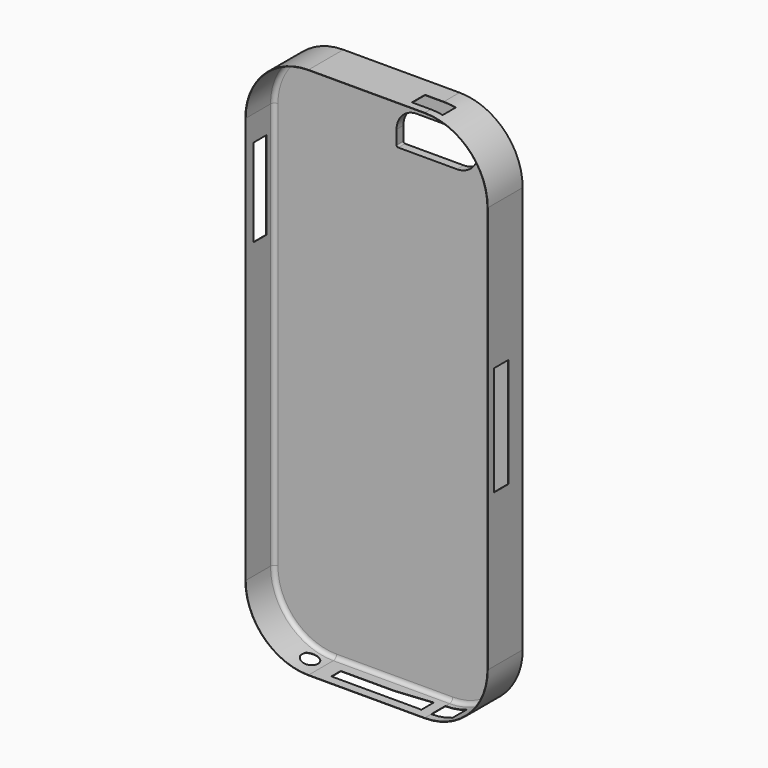
from build123d import *

# Parameters (mm, degrees)
F1_DEPTH  = 218.186
F2_T      = -2
F3_R      = 25.4
F4_W      = 98.1684550643
F4_H      = 539.9262309074
F5_DEPTH  = 25
F6_W      = 115.0492340008
F6_H      = 100.8328720927
F6_W_2    = 74.0123927912
F7_DEPTH  = 25
F8_R      = 49.1963337308
F9_DEPTH  = 25
F10_W     = 113.1808534265
F10_H     = 672.4274903536
F11_DEPTH = 25
F14_DEPTH = 25
F15_DEPTH = 50
F16_DEPTH = 115
F17_W     = 239.6771460772
F17_H     = 1011.9701325893
F18_DEPTH = 50


# Not quite as in the source:
# - a feature names something its author has since deleted; it is built from what else it names


with BuildPart() as f1:
    # F0 (on Front) → F1 (new body)
    with BuildSketch(Plane.XZ):
        with BuildLine():
            Line((345.4135119597, 2072.7365876565), (-369.0884880403, 2072.7365876565))
            ThreePointArc((-369.0884880403, 2072.7365876565), (-643.5251151002, 1959.0612147164), (-757.2004880403, 1684.6245876565))
            Line((-757.2004880403, 1684.6245876565), (-757.2004880403, -817.2754123435))
            ThreePointArc((-757.2004880403, -817.2754123435), (-643.5251151002, -1091.7120394034), (-369.0884880403, -1205.3874123435))
            Line((-369.0884880403, -1205.3874123435), (345.4135119597, -1205.3874123435))
            ThreePointArc((345.4135119597, -1205.3874123435), (619.8501390195, -1091.7120394034), (733.5255119597, -817.2754123435))
            Line((733.5255119597, -817.2754123435), (733.5255119597, 1684.6245876565))
            ThreePointArc((733.5255119597, 1684.6245876565), (619.8501390195, 1959.0612147164), (345.4135119597, 2072.7365876565))
        make_face()
    extrude(amount=F1_DEPTH)

    # F2
    f2_openings = [f1.faces().sort_by_distance(p)[0] for p in [
        (-11.837488, -218.186, 433.674588),
    ]]
    offset(amount=F2_T, openings=f2_openings)

    # F3
    f3_edges = [f1.edges().sort_by_distance(p)[0] for p in [
        (731.525512, -2, 433.674588),
    ]]
    fillet(f3_edges, radius=F3_R)

    # F4 (on face) → F5 (cut)
    with BuildSketch(Plane(origin=(-757.2004880403, 0, 0), x_dir=(0, -1, 0), z_dir=(-1, 0, 0))):
        with Locations((108.4061600268, 1258.9028179646)):
            Rectangle(F4_W, F4_H)
    extrude(amount=-F5_DEPTH, mode=Mode.SUBTRACT)

    # F6 (on face) → F7 (cut)
    with BuildSketch(Plane.XY.offset(2072.7365876565)):
        with Locations((287.8888949593, -121.6761954129)):
            Rectangle(F6_W, F6_H)
        with Locations((382.4197083552, -121.6761954129)):
            Rectangle(F6_W_2, F6_H)
    extrude(amount=-F7_DEPTH, mode=Mode.SUBTRACT)

    # F8 (on face) → F9 (cut)
    with BuildSketch(Plane(origin=(0, 0, -1205.3874123435), x_dir=(1, 0, 0), z_dir=(0, 0, -1))):
        Polygon((254.6437084675, 88.0523696542), (55.4660335183, 88.0523696542), (256.1990016318, 67.995804056), align=None)
        Polygon((254.6437084675, 160.4788154364), (-274.0693688393, 160.4788154364), (-274.0693688393, 88.0523696542), (55.4660335183, 88.0523696542), (254.6437084675, 88.0523696542), align=None)
        Polygon((279.685367193, 162.4769285816), (254.6437084675, 160.4788154364), (254.6437084675, 88.0523696542), (256.1990016318, 67.995804056), (279.685367193, 65.6491251025), align=None)
        Polygon((439.4082129002, 167.7214801311), (345.4135119597, 167.7214801311), (345.4135119597, 59.0817891061), (439.4082129002, 59.0817891061), (588.7299776077, 59.0817891061), (588.7299776077, 167.7214801311), align=None)
        with Locations((-453.6294341087, 100.253932178)):
            Circle(F8_R)
    extrude(amount=-F9_DEPTH, mode=Mode.SUBTRACT)

    # F10 (on face) → F11 (cut)
    with BuildSketch(Plane.YZ.offset(733.5255119597)):
        with Locations((-114.8680560291, 460.3053554893)):
            Rectangle(F10_W, F10_H)
    extrude(amount=-F11_DEPTH, mode=Mode.SUBTRACT)

    # F13 (on face) → F14 (cut)
    with BuildSketch(Plane(origin=(0, 0, 0), x_dir=(-1, 0, 0), z_dir=(0, 1, 0))):
        with BuildLine():
            Line((-123.95587248, 1906.9520282745), (-492.2534132004, 1906.9520282745))
            ThreePointArc((-492.2534132004, 1906.9520282745), (-499.3244810122, 1904.0230960864), (-502.2534132004, 1896.9520282745))
            Line((-502.2534132004, 1896.9520282745), (-502.2534132004, 1818.3750739625))
            ThreePointArc((-502.2534132004, 1818.3750739625), (-463.9013340465, 1725.7849643239), (-371.3112244078, 1687.43288517))
            Line((-371.3112244078, 1687.43288517), (-10, 1687.43288517))
            ThreePointArc((-10, 1687.43288517), (-2.9289321881, 1690.3618173581), (0, 1697.43288517))
            Line((0, 1697.43288517), (0, 1782.9961557945))
            ThreePointArc((0, 1782.9961557945), (-36.3058344815, 1870.646193793), (-123.95587248, 1906.9520282745))
        make_face()
    extrude(amount=-F14_DEPTH, mode=Mode.SUBTRACT)

    # F12 (on face) → F15 (join)
    with BuildSketch(Plane(origin=(0, 0, 0), x_dir=(-1, 0, 0), z_dir=(0, 1, 0))):
        with BuildLine():
            Line((369.0884880403, 2072.7365876565), (-345.4135119597, 2072.7365876565))
            ThreePointArc((-345.4135119597, 2072.7365876565), (-619.8501390195, 1959.0612147164), (-733.5255119597, 1684.6245876565))
            Line((-733.5255119597, 1684.6245876565), (-733.5255119597, -817.2754123435))
            ThreePointArc((-733.5255119597, -817.2754123435), (-619.8501390195, -1091.7120394034), (-345.4135119597, -1205.3874123435))
            Line((-345.4135119597, -1205.3874123435), (369.0884880403, -1205.3874123435))
            ThreePointArc((369.0884880403, -1205.3874123435), (643.5251151002, -1091.7120394034), (757.2004880403, -817.2754123435))
            Line((757.2004880403, -817.2754123435), (757.2004880403, 1684.6245876565))
            ThreePointArc((757.2004880403, 1684.6245876565), (643.5251151002, 1959.0612147164), (369.0884880403, 2072.7365876565))
        make_face()
    extrude(amount=F15_DEPTH)

    # F16 (cut): a face of the model
    f16_faces = [f1.faces().sort_by_distance(p)[0] for p in [
        (250.3551806522, 0, 1797.440656852),
    ]]
    extrude(f16_faces, amount=-F16_DEPTH, mode=Mode.SUBTRACT)

    # F17 (on face) → F18 (cut)
    with BuildSketch(Plane(origin=(0, 50, 0), x_dir=(-1, 0, 0), z_dir=(0, 1, 0))):
        with Locations((-8.1355944276, 57.5146228075)):
            Rectangle(F17_W, F17_H)
    extrude(amount=-F18_DEPTH, mode=Mode.SUBTRACT)


solid = f1.part
